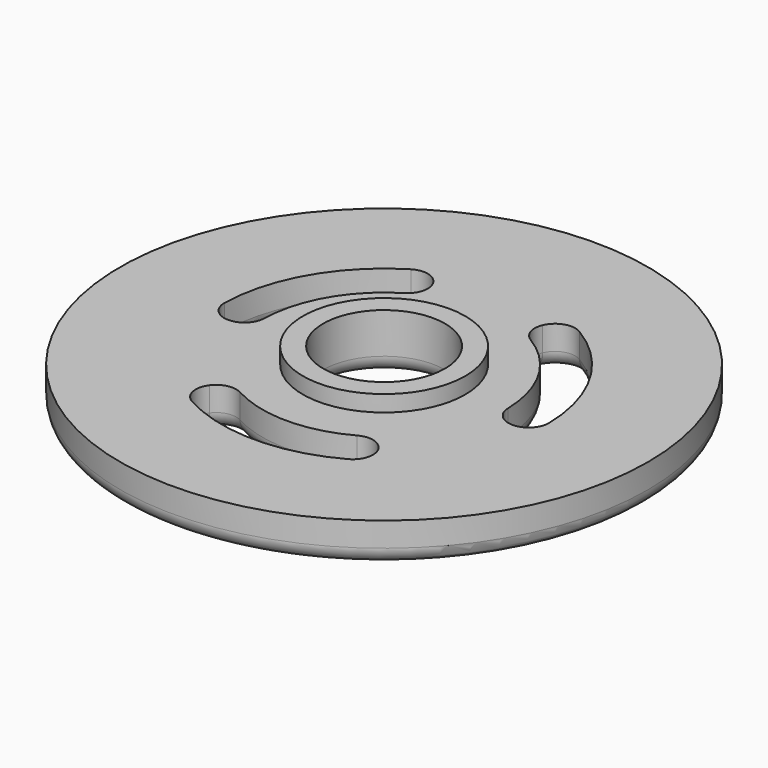
from build123d import *

# Parameters (mm, degrees)
F0_R     = 32.5
F1_DEPTH = 5
F2_R     = 10
F2_R_2   = 7.5
F3_DEPTH = 7
F4_R     = 2


with BuildPart() as f1:
    # F0 (on Top) → F1 (new body)
    with BuildSketch(Plane.XY):
        Circle(F0_R)
        with BuildLine():
            ThreePointArc((-9.6084106433, -17.5407652316), (-10.8510784968, -15.8756509046), (-10.4058874503, -13.8462090975))
            ThreePointArc((-10.4058874503, -13.8462090975), (-8.9348406398, -12.9044503937), (-7.2063079825, -13.1555739237))
            ThreePointArc((-7.2063079825, -13.1555739237), (0, -15), (7.2063079825, -13.1555739237))
            ThreePointArc((7.2063079825, -13.1555739237), (8.9348406398, -12.9044503937), (10.4058874503, -13.8462090975))
            ThreePointArc((10.4058874503, -13.8462090975), (10.8510784968, -15.8756509046), (9.6084106433, -17.5407652316))
            ThreePointArc((9.6084106433, -17.5407652316), (0, -20), (-9.6084106433, -17.5407652316))
        make_face(mode=Mode.SUBTRACT)
        with BuildLine():
            ThreePointArc((-19.994953614, 0.4492549087), (-17.3205080757, 10), (-10.3865429707, 17.0915103229))
            ThreePointArc((-10.3865429707, 17.0915103229), (-8.3231777366, 17.335135089), (-6.7882250994, 15.9348674296))
            ThreePointArc((-6.7882250994, 15.9348674296), (-6.708161543, 14.1900241697), (-7.789907228, 12.8186327422))
            ThreePointArc((-7.789907228, 12.8186327422), (-12.9903810568, 7.5), (-14.9962152105, 0.3369411815))
            ThreePointArc((-14.9962152105, 0.3369411815), (-15.6430021828, -1.285573776), (-17.1941125497, -2.0886583321))
            ThreePointArc((-17.1941125497, -2.0886583321), (-19.1742562334, -1.4594841844), (-19.994953614, 0.4492549087))
        make_face(mode=Mode.SUBTRACT)
        with BuildLine():
            ThreePointArc((0, 10), (7.0710678119, 7.0710678119), (10, 0))
            ThreePointArc((10, 0), (9.6592582629, -2.588190451), (8.6602540378, -5))
            ThreePointArc((8.6602540378, -5), (0, -10), (-8.6602540378, -5))
            ThreePointArc((-8.6602540378, -5), (-8.6602540378, 5), (0, 10))
        make_face(mode=Mode.SUBTRACT)
        with BuildLine():
            ThreePointArc((19.994953614, 0.4492549087), (19.1742562334, -1.4594841844), (17.1941125497, -2.0886583321))
            ThreePointArc((17.1941125497, -2.0886583321), (15.6430021828, -1.285573776), (14.9962152105, 0.3369411815))
            ThreePointArc((14.9962152105, 0.3369411815), (12.9903810568, 7.5), (7.789907228, 12.8186327422))
            ThreePointArc((7.789907228, 12.8186327422), (6.708161543, 14.1900241697), (6.7882250994, 15.9348674296))
            ThreePointArc((6.7882250994, 15.9348674296), (8.3231777366, 17.335135089), (10.3865429707, 17.0915103229))
            ThreePointArc((10.3865429707, 17.0915103229), (17.3205080757, 10), (19.994953614, 0.4492549087))
        make_face(mode=Mode.SUBTRACT)
    extrude(amount=F1_DEPTH)

    # F2 (on face) → F3 (join)
    with BuildSketch(Plane(origin=(0, 0, 0), x_dir=(1, 0, 0), z_dir=(0, 0, -1))):
        Circle(F2_R)
        Circle(F2_R_2, mode=Mode.SUBTRACT)
    extrude(amount=-F3_DEPTH)

    # F4
    f4_edges = [f1.edges().sort_by_distance(p)[0] for p in [
        (-32.5, 0, 0),
        (-10.599955, -14.147118, 0),
        (0, -15, 0),
        (10.599955, -14.147118, 0),
        (0, -20, 0),
        (-17.320508, 10, 0),
        (-6.951786, 16.253389, 0),
        (-12.990381, 7.5, 0),
        (-17.551741, -2.106271, 0),
        (17.551741, -2.106271, 0),
        (12.990381, 7.5, 0),
        (6.951786, 16.253389, 0),
        (17.320508, 10, 0),
        (-7.5, 0, 0),
    ]]
    fillet(f4_edges, radius=F4_R)


solid = f1.part
